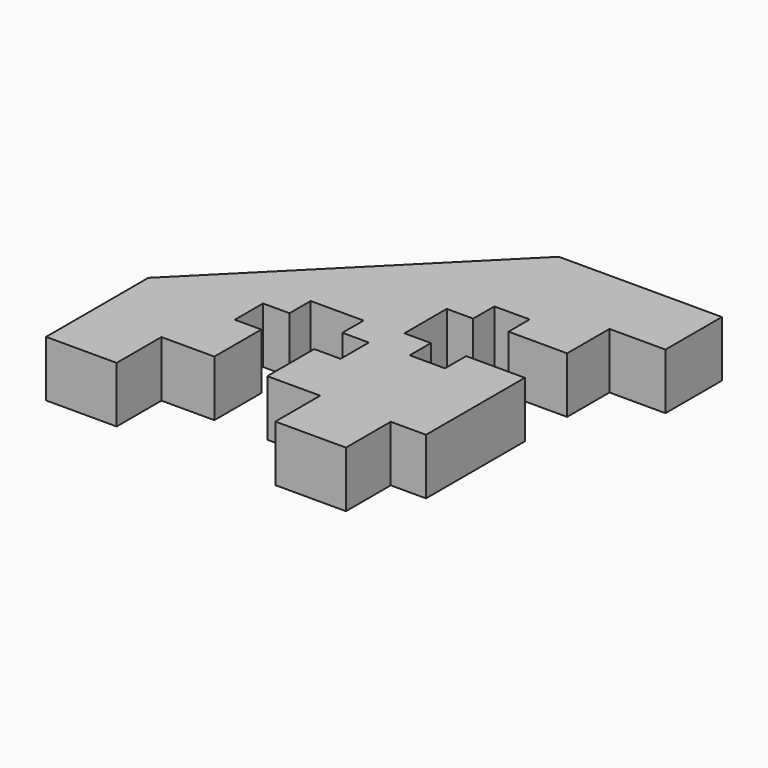
from build123d import *

# Parameters (mm, degrees)
F0_W     = 4
F0_H     = 3.175
F0_W_2   = 3.175
F0_H_2   = 4
F1_DEPTH = 3.175


# Not quite as in the source:
# - a length typed as a fraction of an inch, garbled in the dataset ("3 / 203.2 mm" for 3/8 in), is restored


with BuildPart() as f1:
    # F0 (on Top) → F1 (new body)
    with BuildSketch(Plane.XY):
        Polygon((-25.6521557152, 6.6896411628), (-25.6521557152, 8.1896411628), (-22.6521557152, 8.1896411628), (-22.6521557152, 6.6896411628), (-21.1521557152, 6.6896411628), (-21.1521557152, 4.6896411628), (-22.6521557152, 4.6896411628), (-22.6521557152, 1.3646411628), (-19.6521557152, 1.3646411628), (-15.6521557152, 1.3646411628), (-13.6521557152, 1.3646411628), (-13.6521557152, 5.3646411628), (-13.6521557152, 8.3646411628), (-16.9771557152, 8.3646411628), (-16.9771557152, 6.8646411628), (-18.9771557152, 6.8646411628), (-18.9771557152, 8.3646411628), (-20.4771557152, 8.3646411628), (-20.4771557152, 11.3646411628), (-18.9771557152, 11.3646411628), (-18.9771557152, 12.8646411628), (-16.9771557152, 12.8646411628), (-16.9771557152, 11.3646411628), (-13.6521557152, 11.3646411628), (-13.6521557152, 14.3646411628), (-13.6521557152, 18.3646411628), (-19.7197964023, 18.3646411628), (-32.6521557152, 5.4322818499), (-32.6521557152, 1.3646411628), (-28.6521557152, 1.3646411628), (-25.6521557152, 1.3646411628), (-25.6521557152, 4.6896411628), (-27.1521557152, 4.6896411628), (-27.1521557152, 6.6896411628), align=None)
        with Locations((-30.6521557152, -0.2228588372)):
            Rectangle(F0_W, F0_H)
        with Locations((-17.6521557152, -0.2228588372)):
            Rectangle(F0_W, F0_H)
        with Locations((-12.0646557152, 16.3646411628)):
            Rectangle(F0_W_2, F0_H_2)
    extrude(amount=F1_DEPTH)


solid = f1.part
